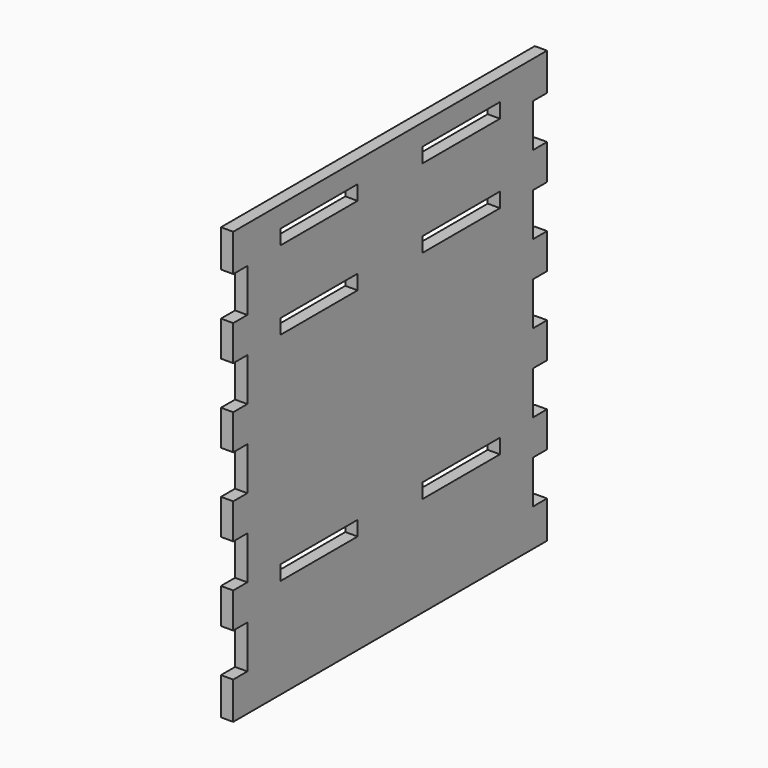
from build123d import *

# Parameters (mm, degrees)
F0_W     = 3.6
F0_H     = 7.6
F0_H_2   = 7.2
F0_W_2   = 19.7
F0_H_3   = 3
F1_DEPTH = 2.5


# Not quite as in the source:
# - a feature names something its author has since deleted; it is built from what else it names


with BuildPart() as f1:
    # F0 (on Right) → F1 (new body)
    with BuildSketch(Plane.YZ):
        with Locations((38.2, -40.2)):
            Rectangle(F0_W, F0_H)
        with Locations((-38.2, -40.2)):
            Rectangle(F0_W, F0_H)
        with Locations((38.2, 40.2)):
            Rectangle(F0_W, F0_H)
        with Locations((-38.2, 40.2)):
            Rectangle(F0_W, F0_H)
        with Locations((38.2, -8)):
            Rectangle(F0_W, F0_H_2)
        with Locations((-38.2, -8)):
            Rectangle(F0_W, F0_H_2)
        Polygon((-36.4, -36.4), (-36.4, -44), (36.4, -44), (36.4, -36.4), (36.4, -27.6), (36.4, -20.4), (36.4, -11.6), (36.4, -4.4), (36.4, 4.4), (36.4, 11.6), (36.4, 20.4), (36.4, 27.6), (36.4, 36.4), (36.4, 44), (-36.4, 44), (-36.4, 36.4), (-36.4, 27.6), (-36.4, 20.4), (-36.4, 11.6), (-36.4, 4.4), (-36.4, -4.4), (-36.4, -11.6), (-36.4, -20.4), (-36.4, -27.6), align=None)
        with Locations((-18.148, -22.104)):
            Rectangle(F0_W_2, F0_H_3, mode=Mode.SUBTRACT)
        with Locations((18.148, -22.104)):
            Rectangle(F0_W_2, F0_H_3, mode=Mode.SUBTRACT)
        with Locations((-18.148, 22.095)):
            Rectangle(F0_W_2, F0_H_3, mode=Mode.SUBTRACT)
        with Locations((-18.148, 38.1555415094)):
            Rectangle(F0_W_2, F0_H_3, mode=Mode.SUBTRACT)
        with Locations((18.148, 22.095)):
            Rectangle(F0_W_2, F0_H_3, mode=Mode.SUBTRACT)
        with Locations((18.148, 38.1555415094)):
            Rectangle(F0_W_2, F0_H_3, mode=Mode.SUBTRACT)
        with Locations((38.2, -24)):
            Rectangle(F0_W, F0_H_2)
        with Locations((-38.2, -24)):
            Rectangle(F0_W, F0_H_2)
        with Locations((38.2, 8)):
            Rectangle(F0_W, F0_H_2)
        with Locations((-38.2, 24)):
            Rectangle(F0_W, F0_H_2)
        with Locations((38.2, 24)):
            Rectangle(F0_W, F0_H_2)
        with Locations((-38.2, 8)):
            Rectangle(F0_W, F0_H_2)
    extrude(amount=F1_DEPTH)


solid = f1.part
